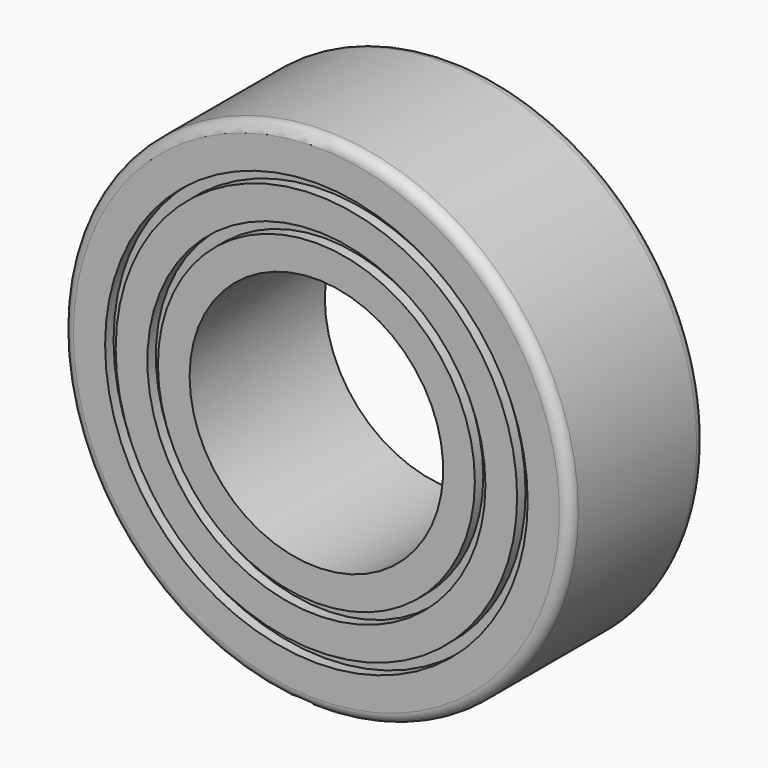
from build123d import *

# Parameters (mm, degrees)
F0_W     = 3
F0_H     = 4
F2_R     = 5
F2_R_2   = 4.75
F2_R_3   = 4
F2_R_4   = 3.75
F3_DEPTH = 0.25
F4_R     = 0.25


# Not quite as in the source:
# - a pattern or mirror of a feature is missing from the dataset's text; its kind, count and spacing are read off the source's solid


with BuildPart() as f1:
    # F0 (on Top) → F1 (revolve)
    with BuildSketch(Plane.XY):
        with Locations((-4.5, 0)):
            Rectangle(F0_W, F0_H)
    revolve(axis=Axis((0, 8.2013355568, 0), (0, 1, 0)))

    # F2 (on face) → F3 (cut)
    with BuildSketch(Plane.XZ.offset(2)):
        Circle(F2_R)
        Circle(F2_R_2, mode=Mode.SUBTRACT)
        Circle(F2_R_3)
        Circle(F2_R_4, mode=Mode.SUBTRACT)
    f3 = extrude(amount=-F3_DEPTH, mode=Mode.SUBTRACT)

    # F3_copies: F3 across plane
    add(f3.mirror(Plane.ZX), mode=Mode.SUBTRACT)

    # F4
    f4_edges = [f1.edges().sort_by_distance(p)[0] for p in [
        (6, -2, 0),
        (6, 2, 0),
    ]]
    fillet(f4_edges, radius=F4_R)


solid = f1.part
